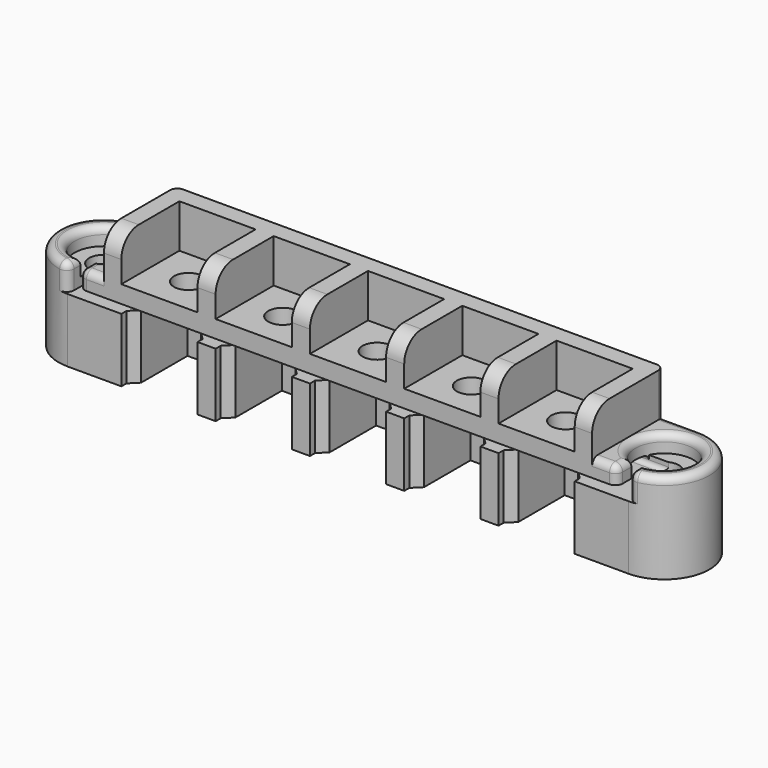
from build123d import *

# Parameters (mm, degrees)
F2_DEPTH      = 10
F3_R          = 2
F4_DEPTH      = 10
F5_W          = 77.3
F5_H          = 1.2
F6_DEPTH      = 8
F8_DEPTH      = 2.4
F10_DEPTH     = 5
F11_R         = 2
F12_DEPTH     = 2.4
F14_DEPTH     = 6
F15_R         = 1
F16_DEPTH     = 2.9
F17_T4_DEPTH  = 16.9595917942
F17_S5_R      = 1
F17_T6_DEPTH  = 10
F17_T10_DEPTH = 16.9595917942
F17_S11_R     = 1
F17_T12_DEPTH = 10
F17_T16_DEPTH = 16.9595917942
F17_S17_R     = 1
F17_T18_DEPTH = 10
F17_T22_DEPTH = 16.9595917942
F17_S23_R     = 1
F17_T24_DEPTH = 10
F17_T28_DEPTH = 16.9595917942
F17_S29_R     = 1
F17_T30_DEPTH = 10
F18_R         = 0.99999
F19_R         = 0.59999
F20_R         = 3
F21_W         = 1.125
F21_H         = 8
F22_DEPTH     = 8.8
F23_SIZE      = 1.12499


# Not quite as in the source:
# - a fillet or chamfer that OpenCascade refuses, or shapes differently, is made with other operations: its cross-section is extruded or revolved along the edge and cut away or added
# - a fillet or chamfer is up to 0.001 mm smaller than in the source, because OpenCascade refuses the exact size


with BuildPart() as f2:
    # F1 (on Top) → F2 (new body)
    with BuildSketch(Plane.XY):
        Polygon((-36.1664630473, 2.4), (-36.1664630473, -10), (-33.7664630473, -10), (-33.7664630473, 0), (-23.2664630473, 0), (-23.2664630473, -10), (-20.7664630473, -10), (-20.7664630473, 0), (-10.2664630473, 0), (-10.2664630473, -10), (-7.7664630473, -10), (-7.7664630473, 0), (2.7335369527, 0), (2.7335369527, -10), (5.2335369527, -10), (5.2335369527, 0), (15.7335369527, 0), (15.7335369527, -10), (18.2335369527, -10), (18.2335369527, 0), (28.7335369527, 0), (28.7335369527, -10), (31.1335369527, -10), (31.1335369527, 2.4), align=None)
    extrude(amount=F2_DEPTH)

    # F3 (on Top) → F4 (join)
    with BuildSketch(Plane.XY):
        with BuildLine():
            Line((-36.1664630473, 2.4), (-41.1664630473, 2.4))
            ThreePointArc((-41.1664630473, 2.4), (-47.3664630473, -3.8), (-41.1664630473, -10))
            Line((-41.1664630473, -10), (-36.1664630473, -10))
            Line((-36.1664630473, -10), (-36.1664630473, 2.4))
        make_face()
        with Locations((-41.1664630473, -3.8)):
            Circle(F3_R, mode=Mode.SUBTRACT)
        with BuildLine():
            ThreePointArc((36.1335369527, -10), (42.3335369527, -3.8), (36.1335369527, 2.4))
            Line((36.1335369527, 2.4), (31.1335369527, 2.4))
            Line((31.1335369527, 2.4), (31.1335369527, -10))
            Line((31.1335369527, -10), (36.1335369527, -10))
        make_face()
        with Locations((36.1335369527, -3.8)):
            Circle(F3_R, mode=Mode.SUBTRACT)
    extrude(amount=F4_DEPTH)

    # F5 (on face) → F6 (cut)
    with BuildSketch(Plane.XZ.offset(10)):
        with Locations((-2.5164630473, 9.4)):
            Rectangle(F5_W, F5_H)
    extrude(amount=-F6_DEPTH, mode=Mode.SUBTRACT)

    # F7 (on face) → F8 (join)
    with BuildSketch(Plane.XY.offset(10)):
        with BuildLine():
            Line((29.8335369527, 2.4), (-36.1664630473, 2.4))
            Line((-36.1664630473, 2.4), (-41.1664630473, 2.4))
            ThreePointArc((-41.1664630473, 2.4), (-47.3664630473, -3.8), (-41.1664630473, -10))
            Line((-41.1664630473, -10), (-36.1664630473, -10))
            Line((-36.1664630473, -10), (29.8335369527, -10))
            Line((29.8335369527, -10), (36.1335369527, -10))
            Line((36.1335369527, -10), (36.1335369527, 2.4))
            Line((36.1335369527, 2.4), (29.8335369527, 2.4))
        make_face()
        with BuildLine():
            ThreePointArc((36.1335369527, -10), (42.3335369527, -3.8), (36.1335369527, 2.4))
            Line((36.1335369527, 2.4), (36.1335369527, -10))
        make_face()
    extrude(amount=F8_DEPTH)

    # F9 (on face) → F10 (cut)
    with BuildSketch(Plane(origin=(0, 0, 10), x_dir=(1, 0, 0), z_dir=(0, 0, -1))):
        with BuildLine():
            Line((-41.1664630473, 10), (-41.1664630473, 7.8))
            ThreePointArc((-41.1664630473, 7.8), (-41.983701622, -0.1156252517), (-39.5664630473, 7.466060556))
            Line((-39.5664630473, 7.466060556), (-39.5664630473, 10))
            Line((-39.5664630473, 10), (-41.1664630473, 10))
        make_face()
        with BuildLine():
            Line((34.5335369527, 10), (34.5335369527, 7.466060556))
            ThreePointArc((34.5335369527, 7.466060556), (36.9507755275, -0.1156252517), (36.1335369527, 7.8))
            Line((36.1335369527, 7.8), (36.1335369527, 10))
            Line((36.1335369527, 10), (34.5335369527, 10))
        make_face()
    extrude(amount=-F10_DEPTH, mode=Mode.SUBTRACT)

    # F11 (on face) → F12 (cut, through all)
    with BuildSketch(Plane.XY.offset(12.4)):
        with Locations((-28.5164630473, -5)):
            Circle(F11_R)
        with Locations((-15.5164630473, -5)):
            Circle(F11_R)
        with Locations((-2.5164630473, -5)):
            Circle(F11_R)
        with Locations((10.4835369527, -5)):
            Circle(F11_R)
        with Locations((23.4835369527, -5)):
            Circle(F11_R)
    extrude(amount=-F12_DEPTH, mode=Mode.SUBTRACT)

    # F13 (on face) → F14 (join)
    with BuildSketch(Plane.XY.offset(12.4)):
        Polygon((-33.7664630473, -10), (-33.7664630473, 0), (-23.2664630473, 0), (-23.2664630473, -10), (-20.7664630473, -10), (-20.7664630473, 0), (-10.2664630473, 0), (-10.2664630473, -10), (-7.7664630473, -10), (-7.7664630473, 0), (2.7335369527, 0), (2.7335369527, -10), (5.2335369527, -10), (5.2335369527, 0), (15.7335369527, 0), (15.7335369527, -10), (18.2335369527, -10), (18.2335369527, 0), (28.7335369527, 0), (28.7335369527, -10), (31.1335369527, -10), (31.1335369527, 2.4), (-36.1664630473, 2.4), (-36.1664630473, -10), align=None)
    extrude(amount=F14_DEPTH)

    # F15 (on face) → F16 (cut)
    with BuildSketch(Plane(origin=(0, 2.4, 0), x_dir=(-1, 0, 0), z_dir=(0, 1, 0))):
        with Locations((-26.5899263322, 12.6)):
            Circle(F15_R)
        with Locations((-13.5899263322, 12.6)):
            Circle(F15_R)
        with Locations((-0.5899263322, 12.6)):
            Circle(F15_R)
        with Locations((12.4100736678, 12.6)):
            Circle(F15_R)
        with Locations((25.4100736678, 12.6)):
            Circle(F15_R)
    extrude(amount=-F16_DEPTH, mode=Mode.SUBTRACT)

    # F17: fillet of radius 3 on 5 edges, made by hand


with BuildPart() as f17_tool2:
    # F17_s3 → F17_t4 (new body)
    with BuildSketch(Plane.YZ.offset(35.0697222293)):
        with BuildLine():
            add(Edge.make_bspline(
                [(-3.5, 12.4), (-0.5, 12.4), (-0.5, 9.4)],
                knots=[0, 0, 0, 1, 1, 1], degree=2, weights=[1, 1, 1]))
            Line((-0.5, 9.4), (-0.5, 12.4))
            Line((-0.5, 12.4), (-3.5, 12.4))
        make_face()
    extrude(amount=-F17_T4_DEPTH)

    # F17_s5 → F17_t6 (intersect, symmetric)
    with BuildSketch(Plane.XZ.offset(2)):
        with Locations((26.5899263322, 12.6)):
            Circle(F17_S5_R)
    extrude(amount=F17_T6_DEPTH, both=True, mode=Mode.INTERSECT)


with BuildPart() as f2_1:
    add(f2.part)

    # F17_t1: cut F17_tool2
    add(f17_tool2.part, mode=Mode.SUBTRACT)


with BuildPart() as f17_tool8:
    # F17_s9 → F17_t10 (new body)
    with BuildSketch(Plane.YZ.offset(22.0697222293)):
        with BuildLine():
            add(Edge.make_bspline(
                [(-3.5, 12.4), (-0.5, 12.4), (-0.5, 9.4)],
                knots=[0, 0, 0, 1, 1, 1], degree=2, weights=[1, 1, 1]))
            Line((-0.5, 9.4), (-0.5, 12.4))
            Line((-0.5, 12.4), (-3.5, 12.4))
        make_face()
    extrude(amount=-F17_T10_DEPTH)

    # F17_s11 → F17_t12 (intersect, symmetric)
    with BuildSketch(Plane.XZ.offset(2)):
        with Locations((13.5899263322, 12.6)):
            Circle(F17_S11_R)
    extrude(amount=F17_T12_DEPTH, both=True, mode=Mode.INTERSECT)


with BuildPart() as f2_2:
    add(f2_1.part)

    # F17_t7: cut F17_tool8
    add(f17_tool8.part, mode=Mode.SUBTRACT)


with BuildPart() as f17_tool14:
    # F17_s15 → F17_t16 (new body)
    with BuildSketch(Plane.YZ.offset(9.0697222293)):
        with BuildLine():
            add(Edge.make_bspline(
                [(-3.5, 12.4), (-0.5, 12.4), (-0.5, 9.4)],
                knots=[0, 0, 0, 1, 1, 1], degree=2, weights=[1, 1, 1]))
            Line((-0.5, 9.4), (-0.5, 12.4))
            Line((-0.5, 12.4), (-3.5, 12.4))
        make_face()
    extrude(amount=-F17_T16_DEPTH)

    # F17_s17 → F17_t18 (intersect, symmetric)
    with BuildSketch(Plane.XZ.offset(2)):
        with Locations((0.5899263322, 12.6)):
            Circle(F17_S17_R)
    extrude(amount=F17_T18_DEPTH, both=True, mode=Mode.INTERSECT)


with BuildPart() as f2_3:
    add(f2_2.part)

    # F17_t13: cut F17_tool14
    add(f17_tool14.part, mode=Mode.SUBTRACT)


with BuildPart() as f17_tool20:
    # F17_s21 → F17_t22 (new body)
    with BuildSketch(Plane.YZ.offset(-3.9302777707)):
        with BuildLine():
            add(Edge.make_bspline(
                [(-3.5, 12.4), (-0.5, 12.4), (-0.5, 9.4)],
                knots=[0, 0, 0, 1, 1, 1], degree=2, weights=[1, 1, 1]))
            Line((-0.5, 9.4), (-0.5, 12.4))
            Line((-0.5, 12.4), (-3.5, 12.4))
        make_face()
    extrude(amount=-F17_T22_DEPTH)

    # F17_s23 → F17_t24 (intersect, symmetric)
    with BuildSketch(Plane.XZ.offset(2)):
        with Locations((-12.4100736678, 12.6)):
            Circle(F17_S23_R)
    extrude(amount=F17_T24_DEPTH, both=True, mode=Mode.INTERSECT)


with BuildPart() as f2_4:
    add(f2_3.part)

    # F17_t19: cut F17_tool20
    add(f17_tool20.part, mode=Mode.SUBTRACT)


with BuildPart() as f17_tool26:
    # F17_s27 → F17_t28 (new body)
    with BuildSketch(Plane.YZ.offset(-16.9302777707)):
        with BuildLine():
            add(Edge.make_bspline(
                [(-3.5, 12.4), (-0.5, 12.4), (-0.5, 9.4)],
                knots=[0, 0, 0, 1, 1, 1], degree=2, weights=[1, 1, 1]))
            Line((-0.5, 9.4), (-0.5, 12.4))
            Line((-0.5, 12.4), (-3.5, 12.4))
        make_face()
    extrude(amount=-F17_T28_DEPTH)

    # F17_s29 → F17_t30 (intersect, symmetric)
    with BuildSketch(Plane.XZ.offset(2)):
        with Locations((-25.4100736678, 12.6)):
            Circle(F17_S29_R)
    extrude(amount=F17_T30_DEPTH, both=True, mode=Mode.INTERSECT)


with BuildPart() as f2_5:
    add(f2_4.part)

    # F17_t25: cut F17_tool26
    add(f17_tool26.part, mode=Mode.SUBTRACT)

    # F18 (radius 1 in the source; OpenCascade refuses exactly that, so slightly less here)
    f18_edges = [f2_5.edges().sort_by_distance(p)[0] for p in [
        (-39.566463, -10, 11.2),
        (-41.166463, -10, 4.4),
        (-41.166463, -10, 10.6),
        (34.533537, -10, 11.2),
        (36.133537, -10, 4.4),
        (36.133537, -10, 10.6),
        (-47.366463, -3.8, 12.4),
        (-38.666463, 2.4, 12.4),
        (-41.983702, 0.115625, 12.4),
        (-37.866463, -10, 12.4),
        (-39.566463, -8.73303, 12.4),
        (42.333537, -3.8, 12.4),
        (33.633537, 2.4, 12.4),
        (36.950776, 0.115625, 12.4),
        (32.833537, -10, 12.4),
        (34.533537, -8.73303, 12.4),
        (36.133537, -8.9, 12.4),
        (-41.166463, -8.9, 12.4),
        (-24.410074, 2.4, 12.6),
        (-11.410074, 2.4, 12.6),
        (1.589926, 2.4, 12.6),
        (14.589926, 2.4, 12.6),
        (27.589926, 2.4, 12.6),
        (31.133537, 2.4, 15.4),
        (-36.166463, 2.4, 15.4),
    ]]
    fillet(f18_edges, radius=F18_R)

    # F19 (radius 0.6 in the source; OpenCascade refuses exactly that, so slightly less here)
    f19_edges = [f2_5.edges().sort_by_distance(p)[0] for p in [
        (-9.016463, -2, 10),
        (-9.016463, -2, 8.8),
        (-22.016463, -2, 8.8),
        (-22.016463, -2, 10),
        (3.983537, -2, 8.8),
        (3.983537, -2, 10),
        (16.983537, -2, 10),
        (16.983537, -2, 8.8),
        (31.997647, -2, 8.8),
        (30.64748, -2, 10),
        (-35.680406, -2, 10),
        (-37.030573, -2, 8.8),
    ]]
    fillet(f19_edges, radius=F19_R)

    # F20
    f20_edges = [f2_5.edges().sort_by_distance(p)[0] for p in [
        (29.933537, -10, 18.4),
        (16.983537, -10, 18.4),
        (3.983537, -10, 18.4),
        (-9.016463, -10, 18.4),
        (-22.016463, -10, 18.4),
        (-34.966463, -10, 18.4),
    ]]
    fillet(f20_edges, radius=F20_R)

    # F21 (on face) → F22 (join)
    with BuildSketch(Plane(origin=(0, 0, 0), x_dir=(1, 0, 0), z_dir=(0, 0, -1))):
        with Locations((28.1710369527, 4)):
            Rectangle(F21_W, F21_H)
        with Locations((18.7960369527, 4)):
            Rectangle(F21_W, F21_H)
        with Locations((5.7960369527, 4)):
            Rectangle(F21_W, F21_H)
        with Locations((15.1710369527, 4)):
            Rectangle(F21_W, F21_H)
        with Locations((-7.2039630473, 4)):
            Rectangle(F21_W, F21_H)
        with Locations((2.1710369527, 4)):
            Rectangle(F21_W, F21_H)
        with Locations((-20.2039630473, 4)):
            Rectangle(F21_W, F21_H)
        with Locations((-10.8289630473, 4)):
            Rectangle(F21_W, F21_H)
        with Locations((-33.2039630473, 4)):
            Rectangle(F21_W, F21_H)
        with Locations((-23.8289630473, 4)):
            Rectangle(F21_W, F21_H)
    extrude(amount=-F22_DEPTH)

    # F23 (size 1.125 in the source; OpenCascade refuses exactly that, so slightly less here)
    f23_edges = [f2_5.edges().sort_by_distance(p)[0] for p in [
        (18.233537, -8, 4.4),
        (28.733537, -8, 4.4),
        (15.733537, -8, 4.4),
        (5.233537, -8, 4.4),
        (-7.766463, -8, 4.4),
        (2.733537, -8, 4.4),
        (-10.266463, -8, 4.4),
        (-23.266463, -8, 4.4),
        (-33.766463, -8, 4.4),
        (-20.766463, -8, 4.4),
    ]]
    chamfer(f23_edges, length=F23_SIZE)


solid = f2_5.part
